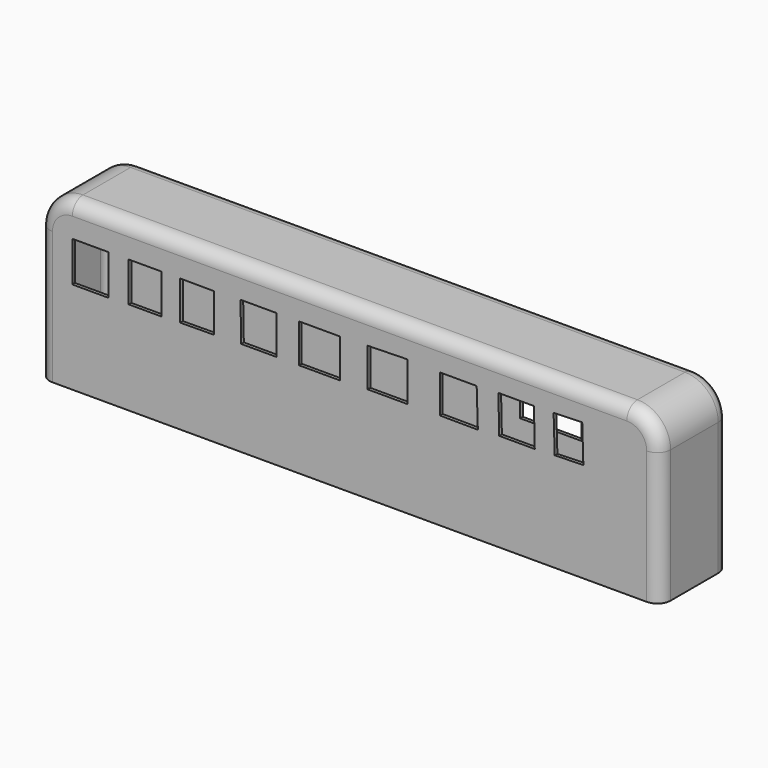
from build123d import *

# Parameters (mm, degrees)
F0_W     = 93.4718027711
F0_H     = 12.9508469254
F1_DEPTH = 25
F2_R     = 5
F3_R     = 5
F4_R     = 2
F5_T     = -0.5
F6_W     = 5.4559892522
F6_H     = 6.0577589622
F6_W_2   = 4.9121007323
F6_H_2   = 5.9622740373
F6_W_3   = 6.1655344907
F6_H_3   = 5.8267693967
F7_DEPTH = 10
F8_W     = 9.2564252019
F8_H     = 7.081441097
F9_DEPTH = 5


with BuildPart() as f1:
    # F0 (on Top) → F1 (new body)
    with BuildSketch(Plane.XY):
        Rectangle(F0_W, F0_H)
    extrude(amount=F1_DEPTH)

    # F2
    f2_edges = [f1.edges().sort_by_distance(p)[0] for p in [
        (46.735901, 0, 25),
    ]]
    fillet(f2_edges, radius=F2_R)

    # F3
    f3_edges = [f1.edges().sort_by_distance(p)[0] for p in [
        (-46.735901, 0, 25),
    ]]
    fillet(f3_edges, radius=F3_R)

    # F4
    f4_edges = [f1.edges().sort_by_distance(p)[0] for p in [
        (0, -6.475423, 25),
        (0, 6.475423, 25),
        (46.735901, 6.475423, 10),
        (46.735901, -6.475423, 10),
        (-46.735901, -6.475423, 10),
        (-45.271435, -6.475423, 23.535534),
        (45.271435, -6.475423, 23.535534),
        (-45.271435, 6.475423, 23.535534),
        (45.271435, 6.475423, 23.535534),
        (-46.735901, 6.475423, 10),
    ]]
    fillet(f4_edges, radius=F4_R)

    # F5
    f5_openings = [f1.faces().sort_by_distance(p)[0] for p in [
        (0, 0, 0),
    ]]
    offset(amount=F5_T, openings=f5_openings)

    # F6 (on face) → F7 (cut)
    with BuildSketch(Plane.XZ.offset(6.4754234627)):
        with Locations((-39.0079067595, 16.9711205189)):
            Rectangle(F6_W, F6_H)
        with Locations((-30.8063998818, 17.0389381237)):
            Rectangle(F6_W_2, F6_H_2)
        Polygon((-25.5047174612, 20.0200751424), (-25.5047174612, 14.1596693691), (-20.3863596622, 14.2051883272), (-20.43789451, 20), align=None)
        Polygon((-16.4258014411, 20.155582577), (-16.3241717964, 14.3288131803), (-10.9716746956, 14.3288131803), (-10.9716746956, 20.155582577), align=None)
        with Locations((-4.5351273147, 17.2421978787)):
            Rectangle(F6_W_3, F6_H_3)
        Polygon((2.711430509, 20.2894311491), (2.711430509, 14.4981949606), (8.747510295, 14.4981949606), (8.747510295, 20.4250746066), align=None)
        Polygon((19.1331994785, 20.2894311491), (13.6082590709, 20.2894311491), (13.6082590709, 14.5744122565), (19.308578223, 14.5405353978), align=None)
        Polygon((22.3996791117, 20.4367674267), (22.5268509239, 14.7776724771), (27.8793480247, 14.7776724771), (27.7521591139, 20.4375283061), align=None)
        Polygon((30.7136761403, 20.5000031751), (30.8842776962, 14.9077031341), (35.1938740726, 15.0391738782), (35.0232725167, 20.6314739191), align=None)
    extrude(amount=-F7_DEPTH, mode=Mode.SUBTRACT)

    # F8 (on face) → F9 (cut)
    with BuildSketch(Plane(origin=(0, 6.4754234627, 0), x_dir=(-1, 0, 0), z_dir=(0, 1, 0))):
        with Locations((-37.1076887846, 16.4592794515)):
            Rectangle(F8_W, F8_H)
        with Locations((-20.3512632847, 13.3706254326)):
            Rectangle(F8_W, F8_H)
    extrude(amount=-F9_DEPTH, mode=Mode.SUBTRACT)


solid = f1.part
